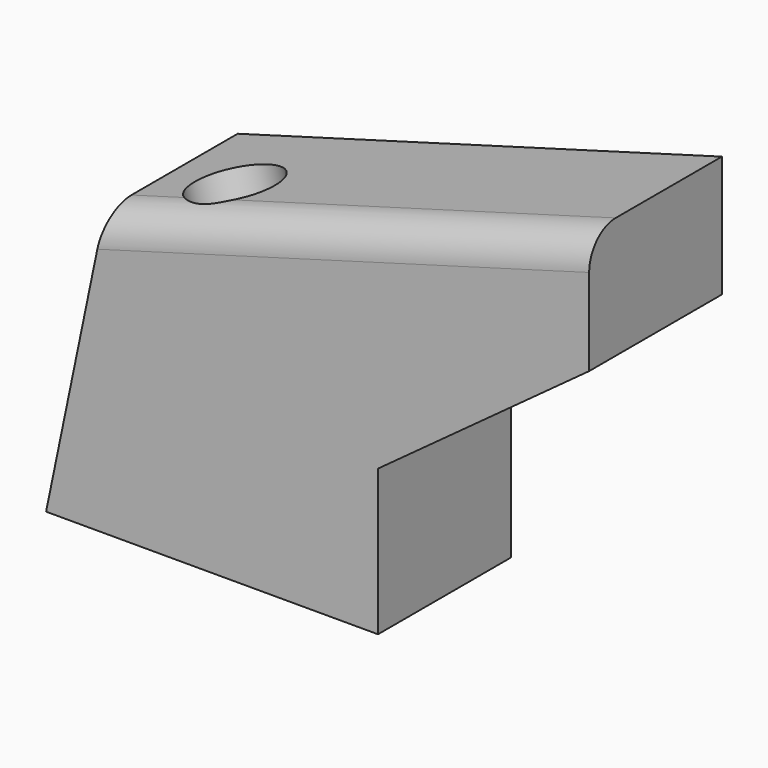
from build123d import *

# Parameters (mm, degrees)
F1_DEPTH    = 25.4
F2_R        = 6.35
F3_DEPTH    = 62.0948563832
F4_T1_DEPTH = 102.4319350424


# Not quite as in the source:
# - a fillet or chamfer that OpenCascade refuses, or shapes differently, is made with other operations: its cross-section is extruded or revolved along the edge and cut away or added


with BuildPart() as f1:
    # F0 (on Front) → F1 (new body)
    with BuildSketch(Plane.XZ):
        Polygon((-12.7767093225, -11.5208044833), (-12.7767093225, 10.8061201186), (19.5394920482, 34.4463924892), (19.5394920482, 53.020893242), (-54.5708905419, 32.0073212298), (-63.5767093225, -11.5208044833), align=None)
    extrude(amount=F1_DEPTH)

    # F2 (on face) → F3 (cut, through all)
    with BuildSketch(Plane(origin=(-12.4610134404, 0, 43.9473342748), x_dir=(0.96207349, 0, 0.2727903953), z_dir=(-0.2727903953, 0, 0.96207349))):
        with Locations((-31.4930230379, -15.3000373393)):
            Circle(F2_R)
    extrude(amount=-F3_DEPTH, mode=Mode.SUBTRACT)

    # F4: fillet of radius 5.08 on 1 edges, made by hand

    # F4_s2 → F4_t1 (cut)
    with BuildSketch(Plane(origin=(44.218838812, 0, 12.5379969877), x_dir=(0, 1, 0), z_dir=(-0.96207349, 0, -0.2727903953))):
        with BuildLine():
            ThreePointArc((-25.4, -40.5998100459), (-23.9121024484, -44.1919124943), (-20.32, -45.6798100459))
            Line((-20.32, -45.6798100459), (-25.4, -45.6798100459))
            Line((-25.4, -45.6798100459), (-25.4, -40.5998100459))
        make_face()
    extrude(amount=F4_T1_DEPTH, mode=Mode.SUBTRACT)


solid = f1.part
